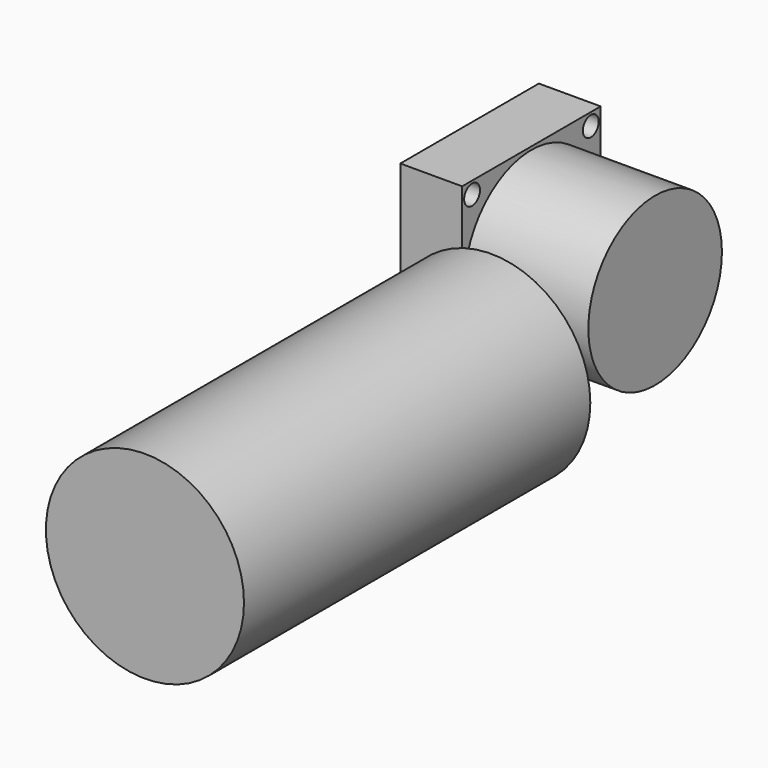
from build123d import *

# Parameters (mm, degrees)
F0_W          = 140
F0_H          = 140
F0_R          = 67.5
F1_DEPTH      = 50
F2_R          = 67.5
F3_DEPTH      = 100
F3_DEPTH_BACK = 25
F4_R          = 8
F5_DEPTH      = 25
F6_R          = 35.981944186
F7_DEPTH      = 100
F8_R          = 80.0728434977
F8_R_2        = 35.981944186
F9_DEPTH      = 350


with BuildPart() as f1:
    # F0 (on Right) → F1 (new body)
    with BuildSketch(Plane.YZ):
        Rectangle(F0_W, F0_H)
        Circle(F0_R, mode=Mode.SUBTRACT)
    extrude(amount=-F1_DEPTH)

    # F4 (on face) → F5 (cut, symmetric)
    with BuildSketch(Plane(origin=(-25, 0, 0), x_dir=(0, -1, 0), z_dir=(-1, 0, 0))):
        with Locations((60, 60)):
            Circle(F4_R)
        with Locations((-60, 60)):
            Circle(F4_R)
        with Locations((-60, -60)):
            Circle(F4_R)
        with Locations((60, -60)):
            Circle(F4_R)
    extrude(amount=F5_DEPTH, both=True, mode=Mode.SUBTRACT)


with BuildPart() as f3:
    # F2 (on face) → F3 (new body, two sides)
    with BuildSketch(Plane.YZ) as f3_sk:
        Circle(F2_R)
    extrude(amount=F3_DEPTH)
    extrude(f3_sk.sketch, amount=-F3_DEPTH_BACK)

    # F6 (on Front) → F7 (join)
    with BuildSketch(Plane.XZ):
        with Locations((47.5254356861, -30.4469484836)):
            Circle(F6_R)
    extrude(amount=F7_DEPTH)

    # F8 (on face) → F9 (join)
    with BuildSketch(Plane.XZ.offset(100)):
        with Locations((47.5254356861, -30.4469484836)):
            Circle(F8_R)
        with Locations((47.5254356861, -30.4469484836)):
            Circle(F8_R_2, mode=Mode.SUBTRACT)
        with Locations((47.5254356861, -30.4469484836)):
            Circle(F8_R_2)
    extrude(amount=F9_DEPTH)


solid = Compound([f1.part, f3.part])
